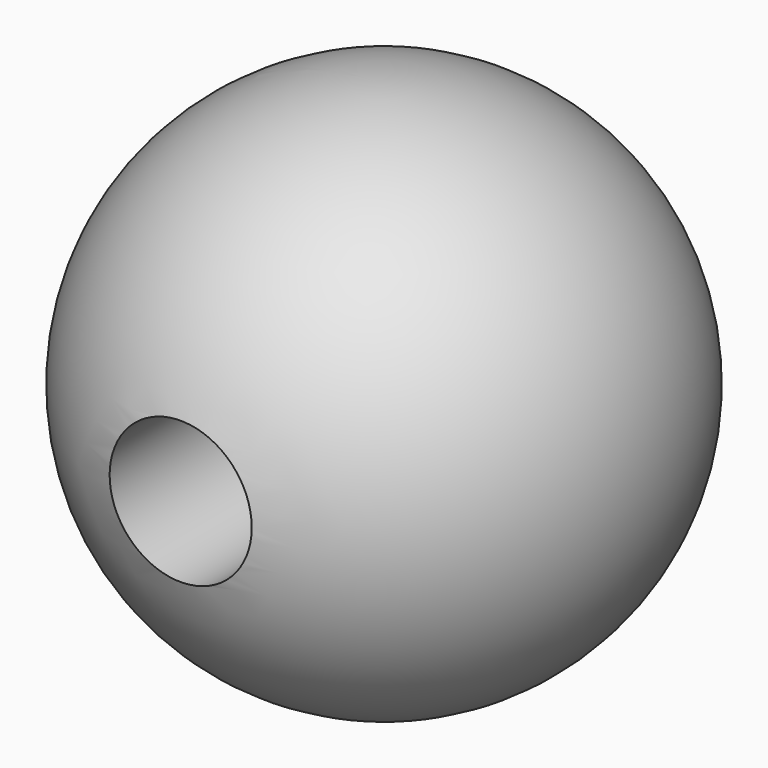
from build123d import *

# Parameters (mm, degrees)
F3_R     = 3.5
F4_DEPTH = 128.4


with BuildPart() as f1:
    # F0 (on Front) → F1 (revolve)
    with BuildSketch(Plane.XZ):
        with BuildLine():
            Line((0, 0), (0, 13))
            ThreePointArc((0, 13), (-13, 0), (0, -13))
            Line((0, -13), (0, 0))
        make_face()
    revolve(axis=Axis((0, 0, -0.8736374089), (0, 0, -1)))

    # F3 (on offset) → F4 (cut)
    with BuildSketch(Plane.XZ.offset(48.5)):
        Circle(F3_R)
    extrude(amount=-F4_DEPTH, mode=Mode.SUBTRACT)


solid = f1.part
